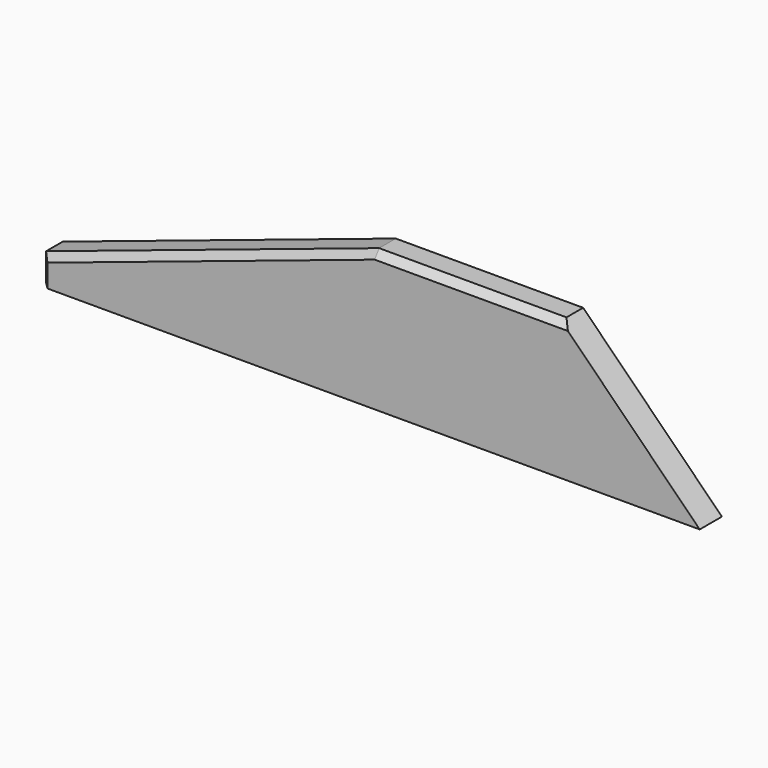
from build123d import *

# Parameters (mm, degrees)
F1_DEPTH = 20
F2_SIZE  = 5
F3_SIZE  = 99.99999


# Not quite as in the source:
# - a fillet or chamfer is up to 0.001 mm smaller than in the source, because OpenCascade refuses the exact size


with BuildPart() as f1:
    # F0 (on Front) → F1 (new body)
    with BuildSketch(Plane.XZ):
        Polygon((-227.9723286629, -18.1198753417), (247.0276713371, -18.1198753417), (247.0276713371, 81.8801246583), (12.0276713371, 81.8801246583), (-227.9723286629, 1.8801246583), align=None)
    extrude(amount=F1_DEPTH)

    # F2
    f2_edges = [f1.edges().sort_by_distance(p)[0] for p in [
        (-107.972329, -20, 41.880125),
        (129.527671, -20, 81.880125),
        (-227.972329, -20, -8.119875),
    ]]
    chamfer(f2_edges, length=F2_SIZE)

    # F3 (size 100 in the source; OpenCascade refuses exactly that, so slightly less here)
    f3_edges = [f1.edges().sort_by_distance(p)[0] for p in [
        (247.027671, -7.5, 81.880125),
    ]]
    chamfer(f3_edges, length=F3_SIZE)


solid = f1.part
